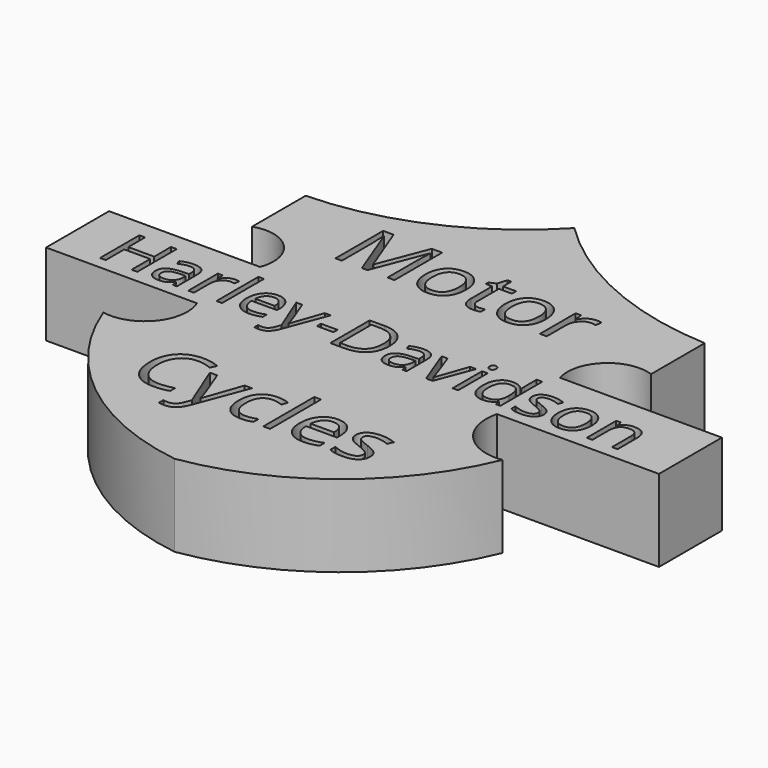
from build123d import *

# Parameters (mm, degrees)
F1_DEPTH       = 12.7
F2_TEXT_SIZE   = 10.6812383617
F2_TEXT_SIZE_2 = 12.9227403603
F2_TEXT_SIZE_3 = 13.0034595107
F3_DEPTH       = 4.7625


# Not quite as in the source:
# - a feature names something its author has since deleted; it is built from what else it names
# - Text() gives the source's letters only with a copy of the font that has no kerning and outlines rounded to 1/6400 em; it was checked with that copy


with BuildPart() as f1:
    # F0 (on Top) → F1 (new body)
    with BuildSketch(Plane.XY):
        with BuildLine():
            ThreePointArc((0, 49.3393465877), (-13.9738033652, 39.4203584503), (-30.6895431131, 35.6470905244))
            Line((-30.6895431131, 35.6470905244), (-30.6895431131, 25.2598598599))
            ThreePointArc((-30.6895431131, 25.2598598599), (-24.5799846212, 23.789218133), (-23.352952674, 17.6261113957))
            Line((-23.352952674, 17.6261113957), (-46.7425361276, 17.6261113957))
            Line((-46.7425361276, 17.6261113957), (-46.7425361276, 5.4296925664))
            Line((-46.7425361276, 5.4296925664), (-23.352952674, 5.4296925664))
            ThreePointArc((-23.352952674, 5.4296925664), (-24.355624715, -1.2357318071), (-30.6895431131, -3.5410975106))
            ThreePointArc((-30.6895431131, -3.5410975106), (-18.6970188833, -20.007224129), (0, -28.092732653))
            ThreePointArc((0, -28.092732653), (18.7984206541, -19.9007600012), (31.1616919935, -3.5410975106))
            ThreePointArc((31.1616919935, -3.5410975106), (24.7479326392, -1.2035277243), (23.1351926923, 5.4296925664))
            Line((23.1351926923, 5.4296925664), (48.243265599, 5.4296925664))
            Line((48.243265599, 5.4296925664), (48.243265599, 17.6261113957))
            Line((48.243265599, 17.6261113957), (23.1351926923, 17.6261113957))
            ThreePointArc((23.1351926923, 17.6261113957), (24.8193778355, 23.8918788195), (31.1616919935, 25.2598598599))
            Line((31.1616919935, 25.2598598599), (31.1616919935, 35.6470905244))
            ThreePointArc((31.1616919935, 35.6470905244), (14.3153805648, 39.6131932456), (0, 49.3393465877))
        make_face()
    extrude(amount=F1_DEPTH)

    # F2 (on face) → F3 (cut)
    with BuildSketch(Plane.XY.offset(12.7)):
        with Locations((-40.9784040805, 7.3576108553)):
            Text('Harley-Davidson', F2_TEXT_SIZE, font='Open Sans', text_align=(TextAlign.LEFT, TextAlign.BOTTOM))
        with Locations((-18.8853735297, 25.0962935388)):
            Text('Motor', F2_TEXT_SIZE_2, font='Open Sans', text_align=(TextAlign.LEFT, TextAlign.BOTTOM))
        with Locations((-18.9911462573, -14.7647988051)):
            Text('Cycles', F2_TEXT_SIZE_3, font='Open Sans', text_align=(TextAlign.LEFT, TextAlign.BOTTOM))
    extrude(amount=-F3_DEPTH, mode=Mode.SUBTRACT)


solid = f1.part
